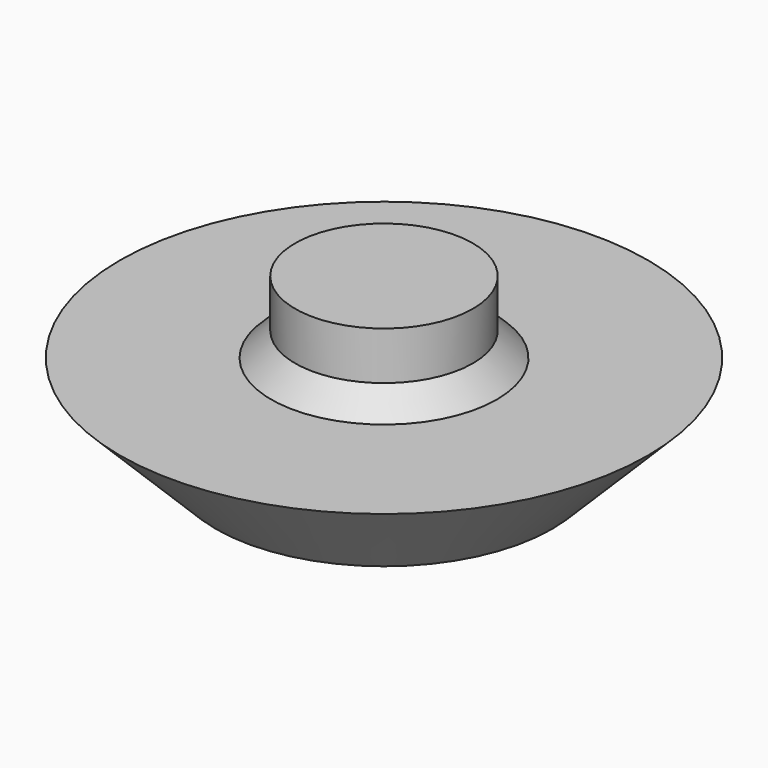
from build123d import *

# Parameters (mm, degrees)
F0_R     = 11
F0_R_2   = 3.7
F1_DEPTH = 4
F2_DEPTH = 7
F3_SIZE  = 3.99999
F4_SIZE  = 1


# Not quite as in the source:
# - a fillet or chamfer is up to 0.001 mm smaller than in the source, because OpenCascade refuses the exact size


with BuildPart() as f1:
    # F0 (on Top) → F1 (new body)
    with BuildSketch(Plane.XY):
        Circle(F0_R)
        Circle(F0_R_2, mode=Mode.SUBTRACT)
        Circle(F0_R_2)
    extrude(amount=F1_DEPTH)

    # F0 (on Top) → F2 (join)
    with BuildSketch(Plane.XY):
        Circle(F0_R_2)
    extrude(amount=F2_DEPTH)

    # F3 (size 4 in the source; OpenCascade refuses exactly that, so slightly less here)
    f3_edges = [f1.edges().sort_by_distance(p)[0] for p in [
        (-11, 0, 0),
    ]]
    chamfer(f3_edges, length=F3_SIZE)

    # F4
    f4_edges = [f1.edges().sort_by_distance(p)[0] for p in [
        (-3.7, 0, 4),
    ]]
    chamfer(f4_edges, length=F4_SIZE)


solid = f1.part
